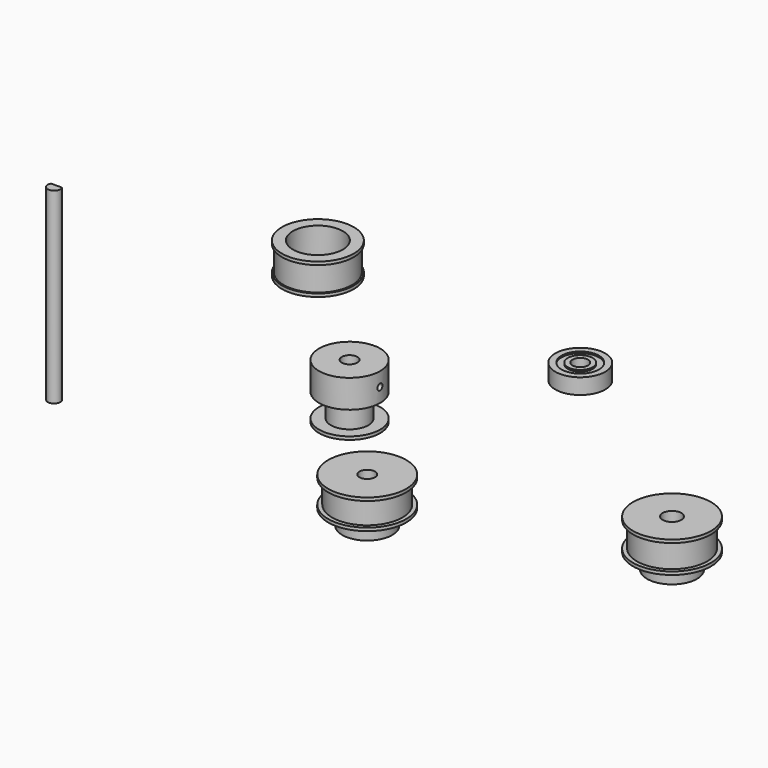
from build123d import *

# Parameters (mm, degrees)
F21_R     = 9.790025198
F21_R_2   = 6
F0_DEPTH  = 9
F1_DEPTH  = 7.5
F22_R     = 9.790025198
F22_R_2   = 6
F2_DEPTH  = 1
F23_DEPTH = 1.5
F3_R      = 2.5
F4_DEPTH  = 18
F5_R      = 11
F5_R_2    = 8
F24_DEPTH = 10
F5_R_3    = 11.5
F25_DEPTH = 1
F26_START = 9
F26_DEPTH = 1
F6_R      = 11.25
F6_R_2    = 8
F6_R_3    = 2.5
F7_DEPTH  = 9.5
F6_R_4    = 12.5
F27_DEPTH = 1
F28_START = 8.5
F28_DEPTH = 1
F8_DEPTH  = 5
F9_R      = 1
F29_DEPTH = 44.5731431246
F11_DEPTH = 10.3096459061
F12_R     = 8
F12_R_2   = 6
F30_DEPTH = 5
F12_R_3   = 4
F12_R_4   = 2.5
F13_START = 0.5
F13_DEPTH = 4
F15_DEPTH = 60
F16_R     = 11.25
F16_R_2   = 8
F16_R_3   = 3
F17_DEPTH = 10
F18_DEPTH = 5
F16_R_4   = 12.5
F19_DEPTH = 1
F20_START = 9
F20_DEPTH = 1


with BuildPart() as f0:
    # F21 (on Top) → F0 (new body)
    with BuildSketch(Plane.XY):
        Circle(F21_R)
        Circle(F21_R_2, mode=Mode.SUBTRACT)
        Circle(F21_R_2)
    extrude(amount=F0_DEPTH)

    # F21 (on Top) → F1 (join)
    with BuildSketch(Plane.XY):
        Circle(F21_R_2)
    extrude(amount=-F1_DEPTH)

    # F22 (on face) → F2 (join)
    with BuildSketch(Plane(origin=(0, 0, -7.5), x_dir=(1, 0, 0), z_dir=(0, 0, -1))):
        Circle(F22_R)
        Circle(F22_R_2, mode=Mode.SUBTRACT)
    extrude(amount=F2_DEPTH)

    # F23 (add): a face of the model
    f23_faces = [f0.faces().sort_by_distance(p)[0] for p in [
        (0, 0, -7.5),
    ]]
    extrude(f23_faces, amount=F23_DEPTH)

    # F3 (on face) → F4 (cut, through all)
    with BuildSketch(Plane(origin=(0, 0, -9), x_dir=(1, 0, 0), z_dir=(0, 0, -1))):
        Circle(F3_R)
    extrude(amount=-F4_DEPTH, mode=Mode.SUBTRACT)

    # F10 (on Right) → F11 (cut)
    with BuildSketch(Plane.YZ):
        with BuildLine():
            ThreePointArc((0.9587933937, 4.5275688171), (0.9352568197, 4.7432518666), (0.865755038, 4.948782036))
            Line((0.865755038, 4.948782036), (-0.9481682506, 4.1063555983))
            ThreePointArc((-0.9481682506, 4.1063555983), (0.1744764432, 3.5511053912), (0.9587933937, 4.5275688171))
        make_face()
        with BuildLine():
            Line((-0.9481682506, 4.1063555983), (0.865755038, 4.948782036))
            ThreePointArc((0.865755038, 4.948782036), (-0.4624198251, 5.4345304615), (-0.9481682506, 4.1063555983))
        make_face()
    extrude(amount=F11_DEPTH, mode=Mode.SUBTRACT)


with BuildPart() as f24:
    # F5 (on Top) → F24 (new body)
    with BuildSketch(Plane.XY):
        with Locations((-45.4013496637, 44.0477058291)):
            Circle(F5_R)
        with Locations((-45.4013496637, 44.0477058291)):
            Circle(F5_R_2, mode=Mode.SUBTRACT)
    extrude(amount=F24_DEPTH)

    # F5 (on Top) → F25 (join)
    with BuildSketch(Plane.XY):
        with Locations((-45.4013496637, 44.0477058291)):
            Circle(F5_R_3)
        with Locations((-45.4013496637, 44.0477058291)):
            Circle(F5_R, mode=Mode.SUBTRACT)
    extrude(amount=F25_DEPTH)

    # F5 (on Top) → F26 (join)
    with BuildSketch(Plane.XY.offset(F26_START)):
        with Locations((-45.4013496637, 44.0477058291)):
            Circle(F5_R_3)
        with Locations((-45.4013496637, 44.0477058291)):
            Circle(F5_R, mode=Mode.SUBTRACT)
    extrude(amount=F26_DEPTH)


with BuildPart() as f7:
    # F6 (on Top) → F7 (new body)
    with BuildSketch(Plane.XY):
        with Locations((42.8172573447, -46.4673861861)):
            Circle(F6_R)
        with Locations((42.8172573447, -46.4673861861)):
            Circle(F6_R_2, mode=Mode.SUBTRACT)
        with Locations((42.8172573447, -46.4673861861)):
            Circle(F6_R_2)
        with Locations((42.8172573447, -46.4673861861)):
            Circle(F6_R_3, mode=Mode.SUBTRACT)
    extrude(amount=F7_DEPTH)

    # F6 (on Top) → F27 (join)
    with BuildSketch(Plane.XY):
        with Locations((42.8172573447, -46.4673861861)):
            Circle(F6_R_4)
        with Locations((42.8172573447, -46.4673861861)):
            Circle(F6_R, mode=Mode.SUBTRACT)
    extrude(amount=F27_DEPTH)

    # F6 (on Top) → F28 (join)
    with BuildSketch(Plane.XY.offset(F28_START)):
        with Locations((42.8172573447, -46.4673861861)):
            Circle(F6_R_4)
        with Locations((42.8172573447, -46.4673861861)):
            Circle(F6_R, mode=Mode.SUBTRACT)
    extrude(amount=F28_DEPTH)

    # F6 (on Top) → F8 (join)
    with BuildSketch(Plane.XY):
        with Locations((42.8172573447, -46.4673861861)):
            Circle(F6_R_2)
        with Locations((42.8172573447, -46.4673861861)):
            Circle(F6_R_3, mode=Mode.SUBTRACT)
    extrude(amount=-F8_DEPTH)

    # F9 (on Front) → F29 (cut)
    with BuildSketch(Plane.XZ):
        with Locations((42.8172573447, -2.5)):
            Circle(F9_R)
    extrude(amount=F29_DEPTH, mode=Mode.SUBTRACT)


with BuildPart() as f30:
    # F12 (on Top) → F30 (new body)
    with BuildSketch(Plane.XY):
        with Locations((41.1711633205, 40.856782347)):
            Circle(F12_R)
        with Locations((41.1711633205, 40.856782347)):
            Circle(F12_R_2, mode=Mode.SUBTRACT)
    extrude(amount=F30_DEPTH)



with BuildPart() as f30b:
    # F12 (on Top) → F30, piece 2 (new body)
    with BuildSketch(Plane.XY):
        with Locations((41.1711633205, 40.856782347)):
            Circle(F12_R_3)
        with Locations((41.1711633205, 40.856782347)):
            Circle(F12_R_4, mode=Mode.SUBTRACT)
    extrude(amount=F30_DEPTH)


with BuildPart() as f30_1:
    add(f30.part)

    add(f30b.part)  # F13 merges F30b
    # F12 (on Top) → F13 (join)
    with BuildSketch(Plane.XY.offset(F13_START)):
        with Locations((41.1711633205, 40.856782347)):
            Circle(F12_R_2)
        with Locations((41.1711633205, 40.856782347)):
            Circle(F12_R_3, mode=Mode.SUBTRACT)
    extrude(amount=F13_DEPTH)


with BuildPart() as f15:
    # F14 (on Top) → F15 (new body)
    with BuildSketch(Plane.XY):
        with BuildLine():
            Line((-53.2196976006, -48.6050862481), (-56.6837992158, -48.6050862481))
            ThreePointArc((-56.6837992158, -48.6050862481), (-54.9517484082, -51.6050862481), (-53.2196976006, -48.6050862481))
        make_face()
    extrude(amount=F15_DEPTH)


with BuildPart() as f17:
    # F16 (on Top) → F17 (new body)
    with BuildSketch(Plane.XY):
        with Locations((117.1524375677, -17.3948351294)):
            Circle(F16_R)
        with Locations((117.1524375677, -17.3948351294)):
            Circle(F16_R_2, mode=Mode.SUBTRACT)
        with Locations((117.1524375677, -17.3948351294)):
            Circle(F16_R_2)
        with Locations((117.1524375677, -17.3948351294)):
            Circle(F16_R_3, mode=Mode.SUBTRACT)
    extrude(amount=F17_DEPTH)

    # F16 (on Top) → F18 (join)
    with BuildSketch(Plane.XY):
        with Locations((117.1524375677, -17.3948351294)):
            Circle(F16_R_2)
        with Locations((117.1524375677, -17.3948351294)):
            Circle(F16_R_3, mode=Mode.SUBTRACT)
    extrude(amount=-F18_DEPTH)

    # F16 (on Top) → F19 (join)
    with BuildSketch(Plane.XY):
        with Locations((117.1524375677, -17.3948351294)):
            Circle(F16_R_4)
        with Locations((117.1524375677, -17.3948351294)):
            Circle(F16_R, mode=Mode.SUBTRACT)
    extrude(amount=F19_DEPTH)

    # F16 (on Top) → F20 (join)
    with BuildSketch(Plane.XY.offset(F20_START)):
        with Locations((117.1524375677, -17.3948351294)):
            Circle(F16_R_4)
        with Locations((117.1524375677, -17.3948351294)):
            Circle(F16_R, mode=Mode.SUBTRACT)
    extrude(amount=F20_DEPTH)


solid = Compound([f0.part, f24.part, f7.part, f30_1.part, f15.part, f17.part])
